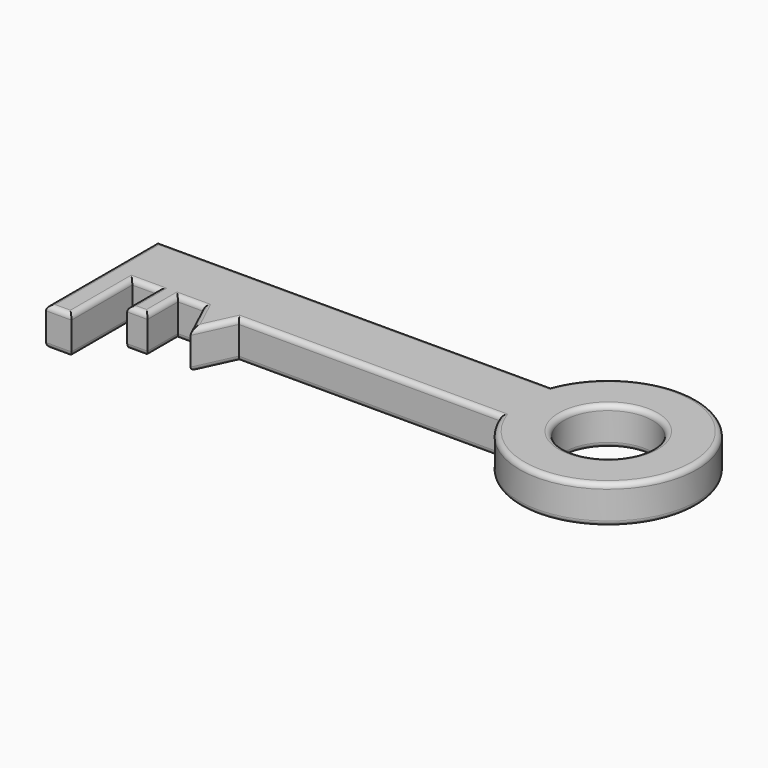
from build123d import *

# Parameters (mm, degrees)
F0_R     = 17.5
F0_W     = 10
F0_H     = 30
F0_W_2   = 8
F0_H_2   = 15
F1_DEPTH = 15
F2_R     = 2
F3_R     = 2


with BuildPart() as f1:
    # F0 (on Top) → F1 (new body)
    with BuildSketch(Plane.XY):
        with BuildLine():
            Line((37.453632827, 21.7892740583), (-117.546367173, 21.7892740583))
            Line((-117.546367173, 21.7892740583), (-117.546367173, -3.2107259417))
            Line((-117.546367173, -3.2107259417), (-107.546367173, -3.2107259417))
            Line((-107.546367173, -3.2107259417), (-97.546367173, -3.2107259417))
            Line((-97.546367173, -3.2107259417), (-89.546367173, -3.2107259417))
            Line((-89.546367173, -3.2107259417), (-79.546367173, -3.2107259417))
            Line((-79.546367173, -3.2107259417), (-65.546367173, -3.2107259417))
            Line((-65.546367173, -3.2107259417), (37.453632827, -3.2107259417))
            ThreePointArc((37.453632827, -3.2107259417), (105.1453749035, 9.2892740583), (37.453632827, 21.7892740583))
        make_face()
        with Locations((70.1453749035, 9.2892740583)):
            Circle(F0_R, mode=Mode.SUBTRACT)
        with Locations((-112.546367173, -18.2107259417)):
            Rectangle(F0_W, F0_H)
        Polygon((-72.546367173, -18.2107862416), (-65.546367173, -3.2107259417), (-79.546367173, -3.2107259417), align=None)
        with Locations((-93.546367173, -10.7107259417)):
            Rectangle(F0_W_2, F0_H_2)
    extrude(amount=F1_DEPTH)

    # F2
    f2_edges = [f1.edges().sort_by_distance(p)[0] for p in [
        (-40.046367, 21.789274, 15),
        (-117.546367, -5.710726, 15),
        (-112.546367, -33.210726, 15),
        (-107.546367, -18.210726, 15),
        (-102.546367, -3.210726, 15),
        (-97.546367, -10.710726, 15),
        (-93.546367, -18.210726, 15),
        (-89.546367, -10.710726, 15),
        (-84.546367, -3.210726, 15),
        (-76.046367, -10.710756, 15),
        (-69.046367, -10.710756, 15),
        (-14.046367, -3.210726, 15),
        (105.145375, 9.289274, 15),
        (52.645375, 9.289274, 15),
    ]]
    fillet(f2_edges, radius=F2_R)

    # F3
    f3_edges = [f1.edges().sort_by_distance(p)[0] for p in [
        (105.145375, 9.289274, 0),
        (52.645375, 9.289274, 0),
        (-40.046367, 21.789274, 0),
        (-14.046367, -3.210726, 0),
        (-69.046367, -10.710756, 0),
        (-89.546367, -10.710726, 0),
        (-93.546367, -18.210726, 0),
        (-107.546367, -18.210726, 0),
        (-117.546367, -5.710726, 0),
        (-112.546367, -33.210726, 0),
        (-102.546367, -3.210726, 0),
        (-76.046367, -10.710756, 0),
        (-84.546367, -3.210726, 0),
    ]]
    fillet(f3_edges, radius=F3_R)


solid = f1.part
